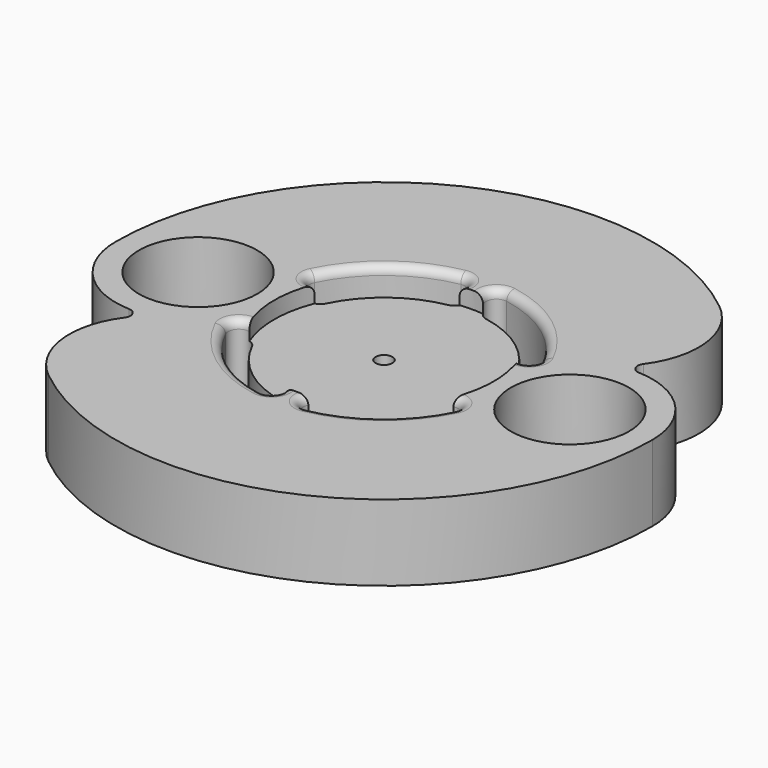
from build123d import *

# Parameters (mm, degrees)
F0_R      = 32.5
F0_R_2    = 7
F0_R_3    = 2.5
F1_DEPTH  = 4.5
F2_R      = 2.5
F2_R_2    = 1
F3_DEPTH  = 6
F4_R      = 32.5
F5_DEPTH  = 5
F6_R      = 13
F7_DEPTH  = 2
F8_DEPTH  = 2
F9_R      = 32.5
F10_DEPTH = 4.001
F12_DEPTH = 9.001
F13_SIZE  = 1.5
F14_R     = 1
F15_R     = 1
F16_SIZE2 = 2.99999
F16_SIZE  = 2.99999


# Not quite as in the source:
# - a fillet or chamfer is up to 0.001 mm smaller than in the source, because OpenCascade refuses the exact size
# - a feature names something its author has since deleted; it is built from what else it names


with BuildPart() as f1:
    # F0 (on Top) → F1 (new body, symmetric)
    with BuildSketch(Plane.XY):
        Circle(F0_R)
        with Locations((-22, 0)):
            Circle(F0_R_2, mode=Mode.SUBTRACT)
        Circle(F0_R_3, mode=Mode.SUBTRACT)
        with Locations((22, 0)):
            Circle(F0_R_2, mode=Mode.SUBTRACT)
    extrude(amount=F1_DEPTH, both=True)

    # F2 (on face) → F3 (join)
    with BuildSketch(Plane.XY.offset(4.5)):
        Circle(F2_R)
        Circle(F2_R_2, mode=Mode.SUBTRACT)
    extrude(amount=-F3_DEPTH)

    # F4 (on face) → F5 (cut)
    with BuildSketch(Plane(origin=(0, 0, -4.5), x_dir=(1, 0, 0), z_dir=(0, 0, -1))):
        Circle(F4_R)
        with BuildLine():
            ThreePointArc((31.75, 0), (28.0826603639, -7.6199568829), (19.8394886364, -9.5076122474))
            ThreePointArc((19.8394886364, -9.5076122474), (23.5322465177, -17.1152835163), (19.8903659997, -24.7474410878))
            ThreePointArc((19.8903659997, -24.7474410878), (-13.7212131298, -28.631989282), (-31.75, 0))
            ThreePointArc((-31.75, 0), (-28.0826603639, 7.6199568829), (-19.8394886364, 9.5076122474))
            ThreePointArc((-19.8394886364, 9.5076122474), (-23.5322465177, 17.1152835163), (-19.8903659997, 24.7474410878))
            ThreePointArc((-19.8903659997, 24.7474410878), (13.7212131298, 28.631989282), (31.75, 0))
        make_face(mode=Mode.SUBTRACT)
    extrude(amount=-F5_DEPTH, mode=Mode.SUBTRACT)

    # F6 (on face) → F7 (cut)
    with BuildSketch(Plane.XY.offset(4.5)):
        Circle(F6_R)
    extrude(amount=-F7_DEPTH, mode=Mode.SUBTRACT)

    # F6 (on face) → F8 (cut)
    with BuildSketch(Plane.XY.offset(4.5)):
        Circle(F6_R)
    extrude(amount=-F8_DEPTH, mode=Mode.SUBTRACT)

    # F9 (on face) → F10 (cut, through all)
    with BuildSketch(Plane(origin=(0, 0, 0.5), x_dir=(1, 0, 0), z_dir=(0, 0, -1))):
        Circle(F9_R)
        with BuildLine():
            ThreePointArc((31.75, 0), (28.0826603639, -7.6199568829), (19.8394886364, -9.5076122474))
            ThreePointArc((19.8394886364, -9.5076122474), (23.5322465177, -17.1152835163), (19.8903659997, -24.7474410878))
            ThreePointArc((19.8903659997, -24.7474410878), (-13.7212131298, -28.631989282), (-31.75, 0))
            ThreePointArc((-31.75, 0), (-28.0826603639, 7.6199568829), (-19.8394886364, 9.5076122474))
            ThreePointArc((-19.8394886364, 9.5076122474), (-23.5322465177, 17.1152835163), (-19.8903659997, 24.7474410878))
            ThreePointArc((-19.8903659997, 24.7474410878), (13.7212131298, 28.631989282), (31.75, 0))
        make_face(mode=Mode.SUBTRACT)
    extrude(amount=-F10_DEPTH, mode=Mode.SUBTRACT)

    # F11 (on face) → F12 (cut, through all)
    with BuildSketch(Plane(origin=(0, 0, -4.5), x_dir=(1, 0, 0), z_dir=(0, 0, -1))):
        with BuildLine():
            ThreePointArc((2.2609964719, -12.2938153132), (1.2577145878, -13.7492964917), (2.7131957663, -14.7525783758))
            ThreePointArc((2.7131957663, -14.7525783758), (9.0657012248, -11.9504418873), (13.4758784029, -6.587920861))
            ThreePointArc((13.4758784029, -6.587920861), (12.9018819411, -4.915937589), (11.2298986691, -5.4899340508))
            ThreePointArc((11.2298986691, -5.4899340508), (7.5547510207, -9.9587015728), (2.2609964719, -12.2938153132))
        make_face()
        with BuildLine():
            ThreePointArc((2.2609964719, 12.2938153132), (7.5547510207, 9.9587015728), (11.2298986691, 5.4899340508))
            ThreePointArc((11.2298986691, 5.4899340508), (12.9018819411, 4.915937589), (13.4758784029, 6.587920861))
            ThreePointArc((13.4758784029, 6.587920861), (9.0657012248, 11.9504418873), (2.7131957663, 14.7525783758))
            ThreePointArc((2.7131957663, 14.7525783758), (1.2577145878, 13.7492964917), (2.2609964719, 12.2938153132))
        make_face()
        with BuildLine():
            ThreePointArc((-13.4758784029, -6.587920861), (-9.0657012248, -11.9504418873), (-2.7131957663, -14.7525783758))
            ThreePointArc((-2.7131957663, -14.7525783758), (-1.2577145878, -13.7492964917), (-2.2609964719, -12.2938153132))
            ThreePointArc((-2.2609964719, -12.2938153132), (-7.5547510207, -9.9587015728), (-11.2298986691, -5.4899340508))
            ThreePointArc((-11.2298986691, -5.4899340508), (-12.9018819411, -4.915937589), (-13.4758784029, -6.587920861))
        make_face()
        with BuildLine():
            ThreePointArc((-11.2271731179, 5.4955057803), (-7.5522799767, 9.9605756437), (-2.2609964719, 12.2938153132))
            ThreePointArc((-2.2609964719, 12.2938153132), (-1.2577145878, 13.7492964917), (-2.7131957663, 14.7525783758))
            ThreePointArc((-2.7131957663, 14.7525783758), (-9.0627359721, 11.9526907724), (-13.4726077415, 6.5946069363))
            ThreePointArc((-13.4726077415, 6.5946069363), (-12.8994410077, 4.9223390465), (-11.2271731179, 5.4955057803))
        make_face()
    extrude(amount=-F12_DEPTH, mode=Mode.SUBTRACT)

    # F13
    f13_edges = [f1.edges().sort_by_distance(p)[0] for p in [
        (15, 0, -4.5),
        (-29, 0, -4.5),
    ]]
    chamfer(f13_edges, length=F13_SIZE)

    # F14
    f14_edges = [f1.edges().sort_by_distance(p)[0] for p in [
        (-19.839489, -9.507612, 0),
        (19.839489, 9.507612, 0),
    ]]
    fillet(f14_edges, radius=F14_R)

    # F15
    f15_edges = [f1.edges().sort_by_distance(p)[0] for p in [
        (-9.065701, 11.950442, 4.5),
        (-9.062736, -11.952691, 4.5),
        (-9.062736, -11.952691, -4.5),
        (9.065701, -11.950442, 4.5),
        (9.065701, -11.950442, -4.5),
        (9.065701, 11.950442, -4.5),
        (9.065701, 11.950442, 4.5),
        (-9.065701, 11.950442, -4.5),
        (1.474921, -14.256683, 4.5),
        (-1.474921, -14.256683, 4.5),
        (13.331976, -5.261826, 4.5),
        (13.331976, 5.261826, 4.5),
        (1.474921, 14.256683, 4.5),
        (-13.329364, -5.26844, 4.5),
        (-13.331976, 5.261826, 4.5),
        (-1.474921, 14.256683, 4.5),
        (12.901882, -4.915938, -4.5),
        (1.257715, -13.749296, -4.5),
        (-1.257715, -13.749296, -4.5),
        (-12.899441, -4.922339, -4.5),
        (-12.901882, 4.915938, -4.5),
        (-1.257715, 13.749296, -4.5),
        (1.257715, 13.749296, -4.5),
        (12.901882, 4.915938, -4.5),
        (-7.55228, -9.960576, -4.5),
        (7.554751, -9.958702, -4.5),
        (-7.554751, 9.958702, -4.5),
        (7.554751, 9.958702, -4.5),
    ]]
    fillet(f15_edges, radius=F15_R)

    # F16 (size 3 and 3 in the source; OpenCascade refuses exactly that, so slightly less here)
    f16_edges = [f1.edges().sort_by_distance(p)[0] for p in [
        (-2.5, 0, -4.5),
    ]]
    chamfer(f16_edges, length=F16_SIZE, length2=F16_SIZE2)


solid = f1.part
